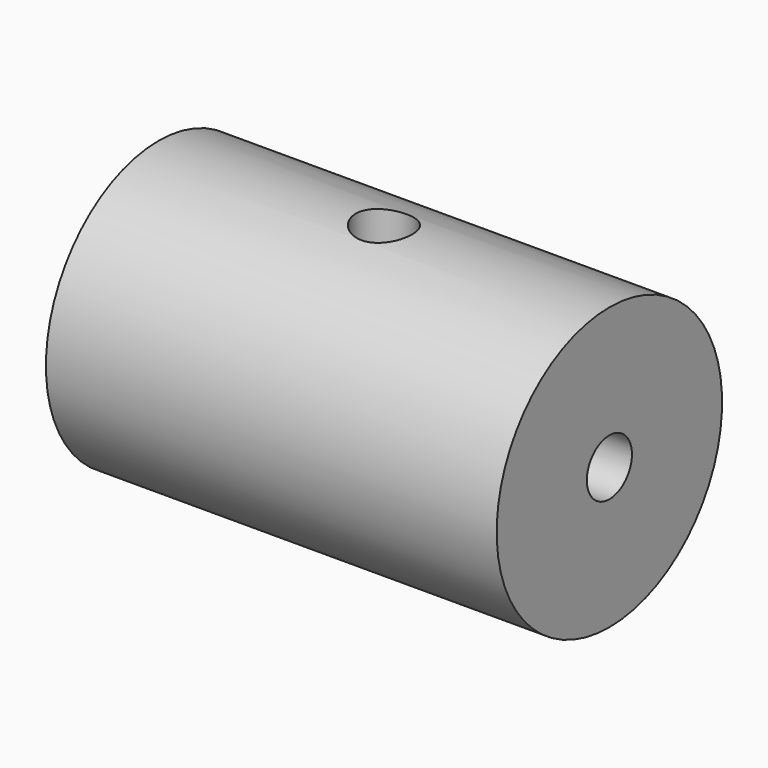
from build123d import *

# Parameters (mm, degrees)
F0_W     = 50.8
F0_H     = 15.875
F2_R     = 3.175
F3_DEPTH = 15.876
F4_R     = 3.175
F5_DEPTH = 50.8010001


# Not quite as in the source:
# - a feature names something its author has since deleted; it is built from what else it names


with BuildPart() as f1:
    # F0 (on Front) → F1 (revolve)
    with BuildSketch(Plane.XZ):
        with Locations((0, 7.9375)):
            Rectangle(F0_W, F0_H)
    revolve(axis=Axis((8.9611150324, 0, 0), (1, 0, 0)))

    # F2 (on Top) → F3 (cut, through all)
    with BuildSketch(Plane.XY):
        Circle(F2_R)
    extrude(amount=F3_DEPTH, mode=Mode.SUBTRACT)

    # F4 (on face) → F5 (cut, through all)
    with BuildSketch(Plane.YZ.offset(25.4)):
        Circle(F4_R)
    extrude(amount=-F5_DEPTH, mode=Mode.SUBTRACT)


solid = f1.part
